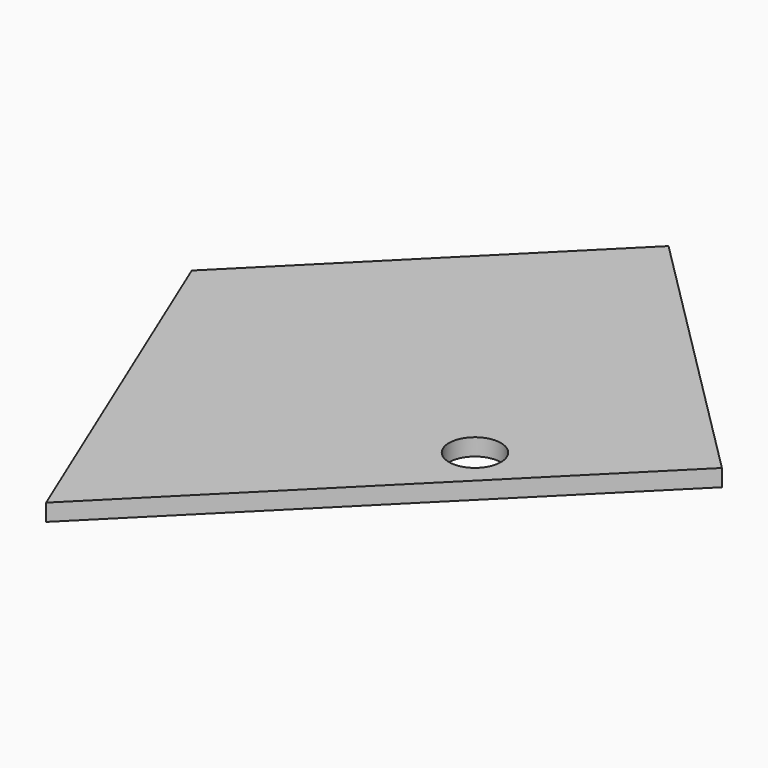
from build123d import *

# Parameters (mm, degrees)
F0_R     = 27.5
F1_DEPTH = 18


with BuildPart() as f1:
    # F0 (on Top) → F1 (new body)
    with BuildSketch(Plane.XY):
        Polygon((1028.858730928, 400), (1194.5441558773, 0), (1592.322943215, 397.7787873377), (1309.4802307404, 680.6214998123), align=None)
        with Locations((1415.5462479183, 291.7127701597)):
            Circle(F0_R, mode=Mode.SUBTRACT)
    extrude(amount=F1_DEPTH)


solid = f1.part
